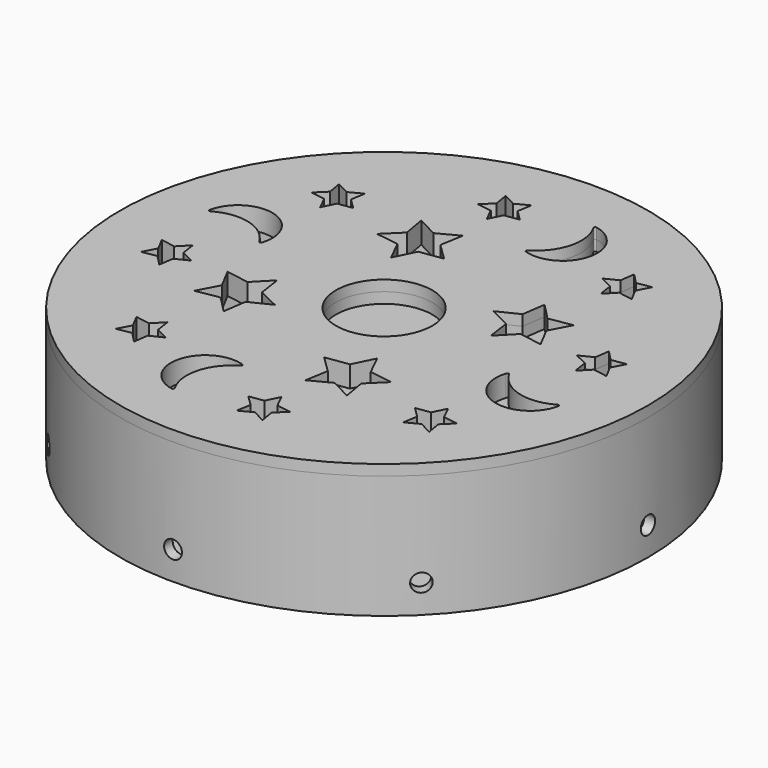
from build123d import *

# Parameters (mm, degrees)
F4_R            = 74
F4_R_2          = 71
F5_DEPTH        = 34.5
F6_DEPTH        = 4.5
F8_R            = 2.5
F9_DEPTH        = 74.001
F9_COPIES_COUNT = 8
F11_W           = 42
F11_H           = 66
F12_DEPTH       = 3
F13_W           = 42
F13_H           = 44
F14_DEPTH       = 1.5
F16_R           = 74
F16_R_2         = 71
F16_R_3         = 70
F16_R_4         = 67
F17_DEPTH       = 3
F18_DEPTH       = 3
F19_R           = 13.5
F20_DEPTH       = 3.001
F20_DEPTH_BACK  = 34.5010001


# Not quite as in the source:
# - a pattern or mirror of a feature is missing from the dataset's text; its kind, count and spacing are read off the source's solid


with BuildPart() as f5:
    # F4 (on Top) → F5 (new body)
    with BuildSketch(Plane.XY):
        Circle(F4_R)
        Circle(F4_R_2, mode=Mode.SUBTRACT)
    extrude(amount=F5_DEPTH)

    # F4 (on Top) → F6 (join)
    with BuildSketch(Plane.XY):
        Circle(F4_R_2)
    extrude(amount=F6_DEPTH)

    # F8 (on Front) → F9 (cut, through all)
    with BuildSketch(Plane.XZ):
        with Locations((0, 8)):
            Circle(F8_R)
    f9 = extrude(amount=-F9_DEPTH, mode=Mode.SUBTRACT)

    # F9_copies: F9 ×8 about axis
    f9_copies_axis = Axis((0, 0, 0), (0, 0, 1))
    for i in range(1, F9_COPIES_COUNT):
        add(f9.rotate(f9_copies_axis, i * 360 / F9_COPIES_COUNT), mode=Mode.SUBTRACT)

    # F11 (on offset) → F12 (cut)
    with BuildSketch(Plane.XY.offset(4.5)):
        with Locations((0, -21)):
            Rectangle(F11_W, F11_H)
    extrude(amount=-F12_DEPTH, mode=Mode.SUBTRACT)

    # F13 (on face) → F14 (join)
    with BuildSketch(Plane.XY.offset(4.5)):
        with Locations((0, -32)):
            Rectangle(F13_W, F13_H)
    extrude(amount=-F14_DEPTH)


with BuildPart() as f17:
    # F16 (on offset) → F17 (new body)
    with BuildSketch(Plane.XY.offset(34.5)):
        Circle(F16_R)
        Circle(F16_R_2, mode=Mode.SUBTRACT)
        Circle(F16_R_2)
        Circle(F16_R_3, mode=Mode.SUBTRACT)
        Circle(F16_R_3)
        Circle(F16_R_4, mode=Mode.SUBTRACT)
        Circle(F16_R_4)
    extrude(amount=F17_DEPTH)

    # F16 (on offset) → F18 (join)
    with BuildSketch(Plane.XY.offset(34.5)):
        Circle(F16_R_3)
        Circle(F16_R_4, mode=Mode.SUBTRACT)
        Circle(F16_R_4)
    extrude(amount=-F18_DEPTH)

    # F19 (on offset) → F20 (cut, two sides)
    with BuildSketch(Plane.XY.offset(34.5)) as f20_sk:
        Polygon((25.5182988048, 16.6654869886), (19.6297549848, 13.7593168765), (25.5182988048, 10.8531467645), (26.4625707148, 4.3547528399), (31.0461628498, 9.0570348582), (37.5182988048, 7.9469766525), (34.4625707148, 13.7593168765), (37.5182988048, 19.5716571006), (31.0461628498, 18.4615988949), (26.4625707148, 23.1638809132), align=None)
        Polygon((50.6721001916, 10.6324617081), (46.9917603041, 8.8161053881), (50.6721001916, 6.9997490681), (51.2622701354, 2.9382528652), (54.1270152197, 5.8771791266), (58.1721001916, 5.1833927481), (56.2622701354, 8.8161053881), (58.1721001916, 12.4488180281), (54.1270152197, 11.7550316495), (51.2622701354, 14.693957911), align=None)
        Polygon((32.2105309231, 42.579320182), (28.5301910356, 40.762963862), (32.2105309231, 38.946607542), (32.8007008668, 34.885111339), (35.6654459512, 37.8240376005), (39.7105309231, 37.1302512219), (37.8007008668, 40.762963862), (39.7105309231, 44.395676502), (35.6654459512, 43.7018901234), (32.8007008668, 46.6408163849), align=None)
        with BuildLine():
            ThreePointArc((7.4648522508, 40.9905597803), (7.2677738003, 40.603083789), (7.5405887992, 40.2646321147))
            ThreePointArc((7.5405887992, 40.2646321147), (19.8787146213, 46.9437063236), (12.5037701828, 58.8789304781))
            ThreePointArc((12.5037701828, 58.8789304781), (12.0986659158, 58.7212342754), (12.0766696729, 58.2870756353))
            ThreePointArc((12.0766696729, 58.2870756353), (13.3480586198, 48.68499303), (7.4648522508, 40.9905597803))
        make_face()
        Circle(F19_R)
        Polygon((-31.0461628498, -18.4615988949), (-26.4625707148, -23.1638809132), (-25.5182988048, -16.6654869886), (-19.6297549848, -13.7593168765), (-25.5182988048, -10.8531467645), (-26.4625707148, -4.3547528399), (-31.0461628498, -9.0570348582), (-37.5182988048, -7.9469766525), (-34.4625707148, -13.7593168765), (-37.5182988048, -19.5716571006), align=None)
        Polygon((-18.4615988949, 31.0461628498), (-23.1638809132, 26.4625707148), (-16.6654869886, 25.5182988048), (-13.7593168765, 19.6297549848), (-10.8531467645, 25.5182988048), (-4.3547528399, 26.4625707148), (-9.0570348582, 31.0461628498), (-7.9469766525, 37.5182988048), (-13.7593168765, 34.4625707148), (-19.5716571006, 37.5182988048), align=None)
        Polygon((-5.1833927481, 58.1721001916), (-8.8161053881, 56.2622701354), (-12.4488180281, 58.1721001916), (-11.7550316495, 54.1270152197), (-14.693957911, 51.2622701354), (-10.6324617081, 50.6721001916), (-8.8161053881, 46.9917603041), (-6.9997490681, 50.6721001916), (-2.9382528652, 51.2622701354), (-5.8771791266, 54.1270152197), align=None)
        Polygon((-40.762963862, 37.8007008668), (-44.395676502, 39.7105309231), (-43.7018901234, 35.6654459512), (-46.6408163849, 32.8007008668), (-42.579320182, 32.2105309231), (-40.762963862, 28.5301910356), (-38.946607542, 32.2105309231), (-34.885111339, 32.8007008668), (-37.8240376005, 35.6654459512), (-37.1302512219, 39.7105309231), align=None)
        Polygon((5.1833927481, -58.1721001916), (8.8161053881, -56.2622701354), (12.4488180281, -58.1721001916), (11.7550316495, -54.1270152197), (14.693957911, -51.2622701354), (10.6324617081, -50.6721001916), (8.8161053881, -46.9917603041), (6.9997490681, -50.6721001916), (2.9382528652, -51.2622701354), (5.8771791266, -54.1270152197), align=None)
        Polygon((40.762963862, -37.8007008668), (44.395676502, -39.7105309231), (43.7018901234, -35.6654459512), (46.6408163849, -32.8007008668), (42.579320182, -32.2105309231), (40.762963862, -28.5301910356), (38.946607542, -32.2105309231), (34.885111339, -32.8007008668), (37.8240376005, -35.6654459512), (37.1302512219, -39.7105309231), align=None)
        Polygon((-37.8007008668, -40.762963862), (-39.7105309231, -44.395676502), (-35.6654459512, -43.7018901234), (-32.8007008668, -46.6408163849), (-32.2105309231, -42.579320182), (-28.5301910356, -40.762963862), (-32.2105309231, -38.946607542), (-32.8007008668, -34.885111339), (-35.6654459512, -37.8240376005), (-39.7105309231, -37.1302512219), align=None)
        Polygon((-58.1721001916, -5.1833927481), (-56.2622701354, -8.8161053881), (-58.1721001916, -12.4488180281), (-54.1270152197, -11.7550316495), (-51.2622701354, -14.693957911), (-50.6721001916, -10.6324617081), (-46.9917603041, -8.8161053881), (-50.6721001916, -6.9997490681), (-51.2622701354, -2.9382528652), (-54.1270152197, -5.8771791266), align=None)
        with BuildLine():
            ThreePointArc((-7.4648522508, -40.9905597803), (-7.2677738003, -40.603083789), (-7.5405887992, -40.2646321147))
            ThreePointArc((-7.5405887992, -40.2646321147), (-19.8787146213, -46.9437063236), (-12.5037701828, -58.8789304781))
            ThreePointArc((-12.5037701828, -58.8789304781), (-12.0986659158, -58.7212342754), (-12.0766696729, -58.2870756353))
            ThreePointArc((-12.0766696729, -58.2870756353), (-13.3480586198, -48.68499303), (-7.4648522508, -40.9905597803))
        make_face()
        with BuildLine():
            ThreePointArc((40.9905597803, -7.4648522508), (40.603083789, -7.2677738003), (40.2646321147, -7.5405887992))
            ThreePointArc((40.2646321147, -7.5405887992), (46.9437063236, -19.8787146213), (58.8789304781, -12.5037701828))
            ThreePointArc((58.8789304781, -12.5037701828), (58.7212342754, -12.0986659158), (58.2870756353, -12.0766696729))
            ThreePointArc((58.2870756353, -12.0766696729), (48.68499303, -13.3480586198), (40.9905597803, -7.4648522508))
        make_face()
        Polygon((18.4615988949, -31.0461628498), (23.1638809132, -26.4625707148), (16.6654869886, -25.5182988048), (13.7593168765, -19.6297549848), (10.8531467645, -25.5182988048), (4.3547528399, -26.4625707148), (9.0570348582, -31.0461628498), (7.9469766525, -37.5182988048), (13.7593168765, -34.4625707148), (19.5716571006, -37.5182988048), align=None)
        with BuildLine():
            ThreePointArc((-40.9905597803, 7.4648522508), (-40.603083789, 7.2677738003), (-40.2646321147, 7.5405887992))
            ThreePointArc((-40.2646321147, 7.5405887992), (-46.9437063236, 19.8787146213), (-58.8789304781, 12.5037701828))
            ThreePointArc((-58.8789304781, 12.5037701828), (-58.7212342754, 12.0986659158), (-58.2870756353, 12.0766696729))
            ThreePointArc((-58.2870756353, 12.0766696729), (-48.68499303, 13.3480586198), (-40.9905597803, 7.4648522508))
        make_face()
    extrude(amount=F20_DEPTH, mode=Mode.SUBTRACT)
    extrude(f20_sk.sketch, amount=-F20_DEPTH_BACK, mode=Mode.SUBTRACT)


solid = Compound([f5.part, f17.part])
